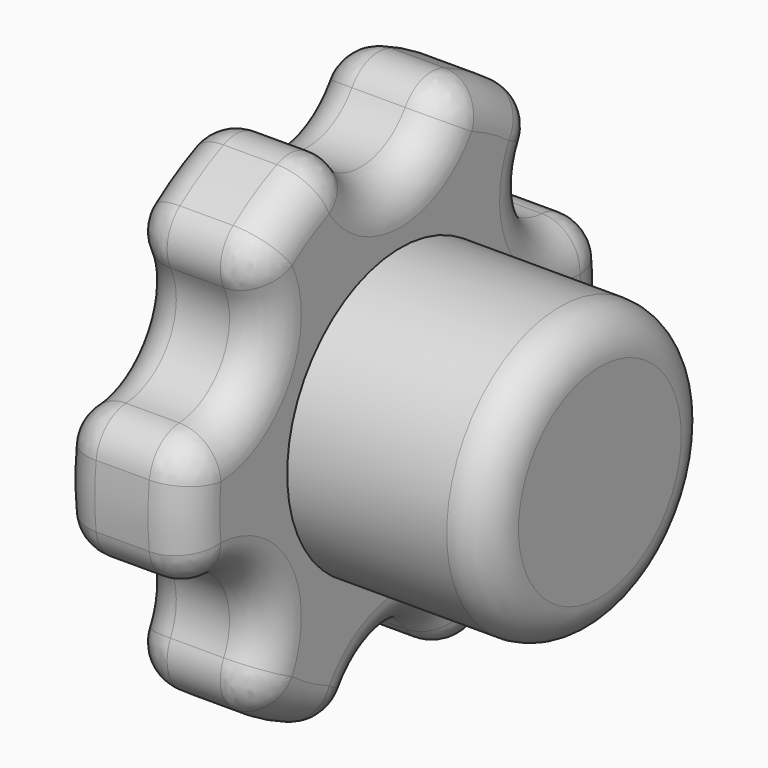
from build123d import *

# Parameters (mm, degrees)
F0_R     = 20
F1_DEPTH = 10
F2_R     = 10.65
F3_DEPTH = 15
F4_R     = 5
F5_DEPTH = 25
F6_R     = 3
F7_R     = 2.999


# Not quite as in the source:
# - two fillets or chamfers of one size are made in one step
# - a fillet or chamfer is up to 0.001 mm smaller than in the source, because OpenCascade refuses the exact size


with BuildPart() as f1:
    # F0 (on Right) → F1 (new body)
    with BuildSketch(Plane.YZ):
        Circle(F0_R)
    extrude(amount=F1_DEPTH)

    # F2 (on face) → F3 (join)
    with BuildSketch(Plane.YZ.offset(10)):
        Circle(F2_R)
    extrude(amount=F3_DEPTH)

    # F4 (on Right) → F5 (cut)
    with BuildSketch(Plane.YZ):
        with Locations((0, 20)):
            Circle(F4_R)
        with Locations((-17.3205080757, 10)):
            Circle(F4_R)
        with Locations((-17.3205080757, -10)):
            Circle(F4_R)
        with Locations((0, -20)):
            Circle(F4_R)
        with Locations((17.3205080757, -10)):
            Circle(F4_R)
        with Locations((17.3205080757, 10)):
            Circle(F4_R)
    extrude(amount=F5_DEPTH, mode=Mode.SUBTRACT)

    # F6
    f6_edges = [f1.edges().sort_by_distance(p)[0] for p in [
        (5, 19.259634, 5.391335),
        (5, 14.29885, 13.983665),
        (5, 4.960784, 19.375),
        (5, -4.960784, 19.375),
        (5, -14.29885, 13.983665),
        (5, -19.259634, 5.391335),
        (5, -19.259634, -5.391335),
        (5, -14.29885, -13.983665),
        (5, -4.960784, -19.375),
        (5, 4.960784, -19.375),
        (5, 19.259634, -5.391335),
        (5, 14.29885, -13.983665),
    ]]
    fillet(f6_edges, radius=F6_R)

    # F7 (radius 3 in the source; OpenCascade refuses exactly that, so slightly less here)
    f7_edges = [f1.edges().sort_by_distance(p)[0] for p in [
        (0, 20, 0),
        (10, 20, 0),
        (0, 18.933295, -4.199813),
        (0, 18.933295, 4.199813),
        (0, 12.990381, -7.5),
        (0, 12.990381, 7.5),
        (0, 13.103793, -14.296808),
        (0, 13.103793, 14.296808),
        (0, 10, -17.320508),
        (0, 10, 17.320508),
        (0, 5.829503, -18.496621),
        (0, 5.829503, 18.496621),
        (0, 0, -15),
        (0, 0, 15),
        (0, -5.829503, -18.496621),
        (0, -5.829503, 18.496621),
        (0, -10, -17.320508),
        (0, -10, 17.320508),
        (0, -13.103793, -14.296808),
        (0, -13.103793, 14.296808),
        (0, -12.990381, -7.5),
        (0, -12.990381, 7.5),
        (0, -18.933295, -4.199813),
        (0, -18.933295, 4.199813),
        (0, -20, 0),
        (10, 18.933295, -4.199813),
        (10, 18.933295, 4.199813),
        (10, 12.990381, -7.5),
        (10, 13.103793, -14.296808),
        (10, 10, -17.320508),
        (10, 5.829503, -18.496621),
        (10, 0, -15),
        (10, 12.990381, 7.5),
        (10, -5.829503, -18.496621),
        (10, 13.103793, 14.296808),
        (10, -10, -17.320508),
        (10, 10, 17.320508),
        (10, -13.103793, -14.296808),
        (10, 5.829503, 18.496621),
        (10, -12.990381, -7.5),
        (10, 0, 15),
        (10, -18.933295, -4.199813),
        (10, -5.829503, 18.496621),
        (10, -20, 0),
        (10, -10, 17.320508),
        (10, -18.933295, 4.199813),
        (10, -13.103793, 14.296808),
        (10, -12.990381, 7.5),
        (25, -10.65, 0),
    ]]
    fillet(f7_edges, radius=F7_R)


solid = f1.part
